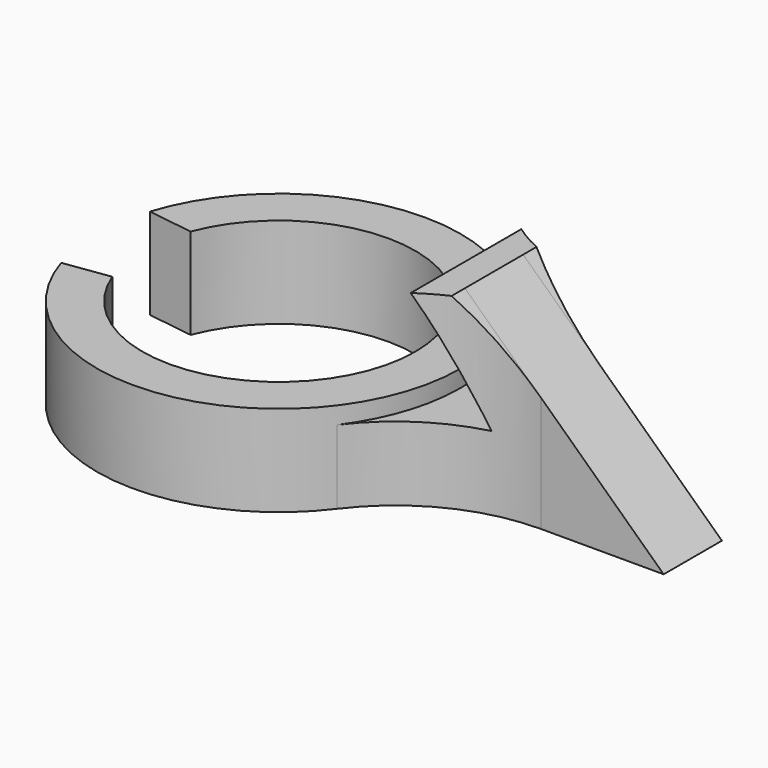
from build123d import *

# Parameters (mm, degrees)
F0_R          = 12.7
F0_R_2        = 9.525
F2_DEPTH      = 6.35
F4_DEPTH      = 25.4
F6_DEPTH      = 2.54
F6_DEPTH_BACK = 2.54
F7_T4_DEPTH   = 24.8484443303
F7_T12_DEPTH  = 24.8484443303
F7_T19_DEPTH  = 5.1569640636
F7_T24_DEPTH  = 5.1569640636
F8_T4_DEPTH   = 24.8484443303
F8_T12_DEPTH  = 24.8484443303
F8_T19_DEPTH  = 5.1569640636
F8_T24_DEPTH  = 5.1569640636


# Not quite as in the source:
# - a fillet or chamfer that OpenCascade refuses, or shapes differently, is made with other operations: its cross-section is extruded or revolved along the edge and cut away or added


with BuildPart() as f2:
    # F0 (on Top) → F2 (new body)
    with BuildSketch(Plane.XY):
        Circle(F0_R)
        Circle(F0_R_2, mode=Mode.SUBTRACT)
    extrude(amount=F2_DEPTH)

    # F3 (on face) → F4 (cut)
    with BuildSketch(Plane.XY.offset(6.35)):
        with BuildLine():
            Line((2.0157811232, 1.8745124225), (-12.0961464615, 3.8695272039))
            ThreePointArc((-12.0961464615, 3.8695272039), (-12.7, 0), (-12.0961464615, -3.8695272039))
            Line((-12.0961464615, -3.8695272039), (2.0157811232, -1.8745124225))
            Line((2.0157811232, -1.8745124225), (2.0157811232, 1.8745124225))
        make_face()
    extrude(amount=-F4_DEPTH, mode=Mode.SUBTRACT)

    # F5 (on Front) → F6 (join, two sides)
    with BuildSketch(Plane.XZ) as f6_sk:
        Polygon((10.5609930441, 5.1569640636), (10.7068819925, 0), (28.8828521035, 0), (15.0134566239, 13.0622601137), (13.0563958547, 13.0622601137), (17.1839392743, 5.1569640636), align=None)
    extrude(amount=F6_DEPTH)
    extrude(f6_sk.sketch, amount=-F6_DEPTH_BACK)

    # F7: fillet of radius 12.7 on 1 edges, made by hand


with BuildPart() as f7_tool2:
    # F7_s3 → F7_t4 (new body)
    with BuildSketch(Plane.XY.offset(24.8484443303)):
        with BuildLine():
            ThreePointArc((10.16, -7.62), (14.6403873372, -3.8807746743), (20.32, -2.54))
            Line((20.32, -2.54), (12.4434078933, -2.54))
            ThreePointArc((12.4434078933, -2.54), (11.5836139481, -5.206715654), (10.16, -7.62))
        make_face()
    extrude(amount=-F7_T4_DEPTH)

    split(bisect_by=Plane.XY.offset(6.35), keep=Keep.TOP)

    split(bisect_by=Plane(origin=(15.6186590558, 0, 8.1548740238), x_dir=(0, 1, 0), z_dir=(0.8864449555, 0, 0.4628340317)), keep=Keep.TOP)

    split(bisect_by=Plane.XY.offset(13.0622601137), keep=Keep.BOTTOM)

    split(bisect_by=Plane(origin=(13.5765905704, 0, 14.4155071364), x_dir=(0, 1, 0), z_dir=(-0.6856071252, 0, -0.7279717507)), keep=Keep.TOP)


with BuildPart() as f2_1:
    add(f2.part)

    # F7_t1: union F7_tool2
    add(f7_tool2.part)


with BuildPart() as f7_tool10:
    # F7_s11 → F7_t12 (new body)
    with BuildSketch(Plane.XY.offset(24.8484443303)):
        with BuildLine():
            ThreePointArc((10.16, -7.62), (14.6403873372, -3.8807746743), (20.32, -2.54))
            Line((20.32, -2.54), (12.4434078933, -2.54))
            ThreePointArc((12.4434078933, -2.54), (11.5836139481, -5.206715654), (10.16, -7.62))
        make_face()
    extrude(amount=-F7_T12_DEPTH)

    split(bisect_by=Plane.XY.offset(5.1569640636), keep=Keep.TOP)

    split(bisect_by=Plane.XY.offset(6.35), keep=Keep.BOTTOM)

    split(bisect_by=Plane(origin=(15.6186590558, 0, 8.1548740238), x_dir=(0, 1, 0), z_dir=(0.8864449555, 0, 0.4628340317)), keep=Keep.TOP)


with BuildPart() as f2_2:
    add(f2_1.part)

    # F7_t9: union F7_tool10
    add(f7_tool10.part)


with BuildPart() as f7_tool17:
    # F7_s18 → F7_t19 (new body)
    with BuildSketch(Plane.XY.offset(5.1569640636)):
        with BuildLine():
            ThreePointArc((10.16, -7.62), (14.6403873372, -3.8807746743), (20.32, -2.54))
            Line((20.32, -2.54), (12.4434078933, -2.54))
            ThreePointArc((12.4434078933, -2.54), (11.5836139481, -5.206715654), (10.16, -7.62))
        make_face()
    extrude(amount=-F7_T19_DEPTH)

    split(bisect_by=Plane(origin=(15.6186590558, 0, 8.1548740238), x_dir=(0, 1, 0), z_dir=(0.8864449555, 0, 0.4628340317)), keep=Keep.TOP)


with BuildPart() as f2_3:
    add(f2_2.part)

    # F7_t16: union F7_tool17
    add(f7_tool17.part)


with BuildPart() as f7_tool22:
    # F7_s23 → F7_t24 (new body)
    with BuildSketch(Plane.XY.offset(5.1569640636)):
        with BuildLine():
            ThreePointArc((10.16, -7.62), (14.6403873372, -3.8807746743), (20.32, -2.54))
            Line((20.32, -2.54), (12.4434078933, -2.54))
            ThreePointArc((12.4434078933, -2.54), (11.5836139481, -5.206715654), (10.16, -7.62))
        make_face()
    extrude(amount=-F7_T24_DEPTH)

    split(bisect_by=Plane(origin=(15.6186590558, 0, 8.1548740238), x_dir=(0, 1, 0), z_dir=(-0.8864449555, 0, -0.4628340317)), keep=Keep.TOP)


with BuildPart() as f2_4:
    add(f2_3.part)

    # F7_t21: union F7_tool22
    add(f7_tool22.part)

    # F8: fillet of radius 12.7 on 1 edges, made by hand


with BuildPart() as f8_tool2:
    # F8_s3 → F8_t4 (new body)
    with BuildSketch(Plane.XY.offset(24.8484443303)):
        with BuildLine():
            ThreePointArc((10.16, 7.62), (14.6403873372, 3.8807746743), (20.32, 2.54))
            Line((20.32, 2.54), (12.4434078933, 2.54))
            ThreePointArc((12.4434078933, 2.54), (11.5836139481, 5.206715654), (10.16, 7.62))
        make_face()
    extrude(amount=-F8_T4_DEPTH)

    split(bisect_by=Plane.XY.offset(6.35), keep=Keep.TOP)

    split(bisect_by=Plane(origin=(15.6186590558, 0, 8.1548740238), x_dir=(0, 1, 0), z_dir=(0.8864449555, 0, 0.4628340317)), keep=Keep.TOP)

    split(bisect_by=Plane.XY.offset(13.0622601137), keep=Keep.BOTTOM)

    split(bisect_by=Plane(origin=(13.5765905704, 0, 14.4155071364), x_dir=(0, 1, 0), z_dir=(-0.6856071252, 0, -0.7279717507)), keep=Keep.TOP)


with BuildPart() as f2_5:
    add(f2_4.part)

    # F8_t1: union F8_tool2
    add(f8_tool2.part)


with BuildPart() as f8_tool10:
    # F8_s11 → F8_t12 (new body)
    with BuildSketch(Plane.XY.offset(24.8484443303)):
        with BuildLine():
            ThreePointArc((10.16, 7.62), (14.6403873372, 3.8807746743), (20.32, 2.54))
            Line((20.32, 2.54), (12.4434078933, 2.54))
            ThreePointArc((12.4434078933, 2.54), (11.5836139481, 5.206715654), (10.16, 7.62))
        make_face()
    extrude(amount=-F8_T12_DEPTH)

    split(bisect_by=Plane.XY.offset(5.1569640636), keep=Keep.TOP)

    split(bisect_by=Plane.XY.offset(6.35), keep=Keep.BOTTOM)

    split(bisect_by=Plane(origin=(15.6186590558, 0, 8.1548740238), x_dir=(0, 1, 0), z_dir=(0.8864449555, 0, 0.4628340317)), keep=Keep.TOP)


with BuildPart() as f2_6:
    add(f2_5.part)

    # F8_t9: union F8_tool10
    add(f8_tool10.part)


with BuildPart() as f8_tool17:
    # F8_s18 → F8_t19 (new body)
    with BuildSketch(Plane.XY.offset(5.1569640636)):
        with BuildLine():
            ThreePointArc((10.16, 7.62), (14.6403873372, 3.8807746743), (20.32, 2.54))
            Line((20.32, 2.54), (12.4434078933, 2.54))
            ThreePointArc((12.4434078933, 2.54), (11.5836139481, 5.206715654), (10.16, 7.62))
        make_face()
    extrude(amount=-F8_T19_DEPTH)

    split(bisect_by=Plane(origin=(15.6186590558, 0, 8.1548740238), x_dir=(0, 1, 0), z_dir=(0.8864449555, 0, 0.4628340317)), keep=Keep.TOP)


with BuildPart() as f2_7:
    add(f2_6.part)

    # F8_t16: union F8_tool17
    add(f8_tool17.part)


with BuildPart() as f8_tool22:
    # F8_s23 → F8_t24 (new body)
    with BuildSketch(Plane.XY.offset(5.1569640636)):
        with BuildLine():
            ThreePointArc((10.16, 7.62), (14.6403873372, 3.8807746743), (20.32, 2.54))
            Line((20.32, 2.54), (12.4434078933, 2.54))
            ThreePointArc((12.4434078933, 2.54), (11.5836139481, 5.206715654), (10.16, 7.62))
        make_face()
    extrude(amount=-F8_T24_DEPTH)

    split(bisect_by=Plane(origin=(15.6186590558, 0, 8.1548740238), x_dir=(0, 1, 0), z_dir=(-0.8864449555, 0, -0.4628340317)), keep=Keep.TOP)


with BuildPart() as f2_8:
    add(f2_7.part)

    # F8_t21: union F8_tool22
    add(f8_tool22.part)


solid = f2_8.part
